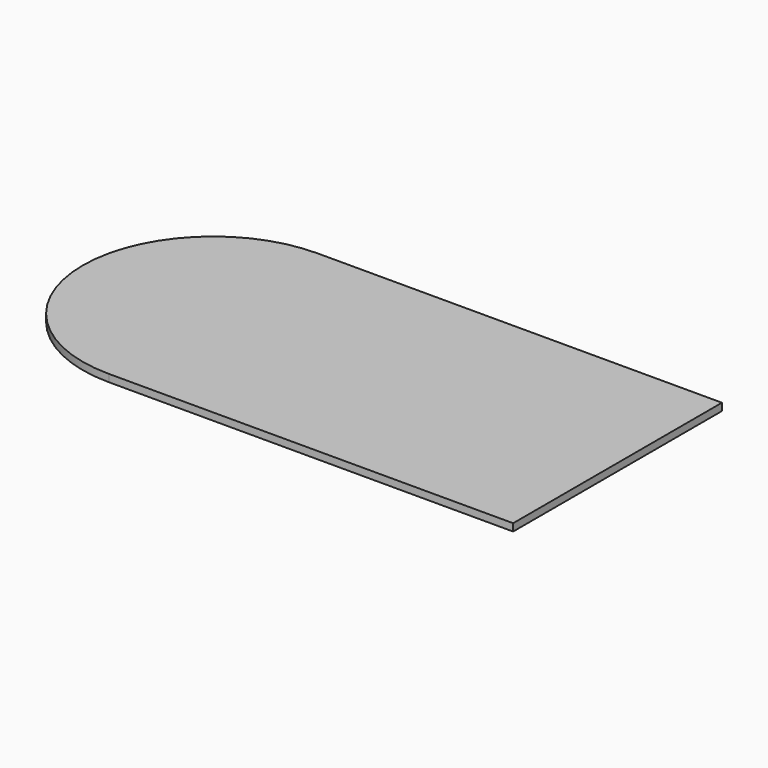
from build123d import *

# Parameters (mm, degrees)
F1_DEPTH = 1


with BuildPart() as f1:
    # F0 (on Top) → F1 (new body)
    with BuildSketch(Plane.XY):
        with BuildLine():
            ThreePointArc((0, -17.75), (12.5511453661, -12.5511453661), (17.75, 0))
            ThreePointArc((17.75, 0), (12.5511453661, 12.5511453661), (0, 17.75))
            ThreePointArc((0, 17.75), (-17.75, 0), (0, -17.75))
        make_face()
        with BuildLine():
            ThreePointArc((0, 17.75), (12.5511453661, 12.5511453661), (17.75, 0))
            ThreePointArc((17.75, 0), (12.5511453661, -12.5511453661), (0, -17.75))
            Line((0, -17.75), (55, -17.75))
            Line((55, -17.75), (55, 17.75))
            Line((55, 17.75), (0, 17.75))
        make_face()
    extrude(amount=F1_DEPTH)


solid = f1.part
